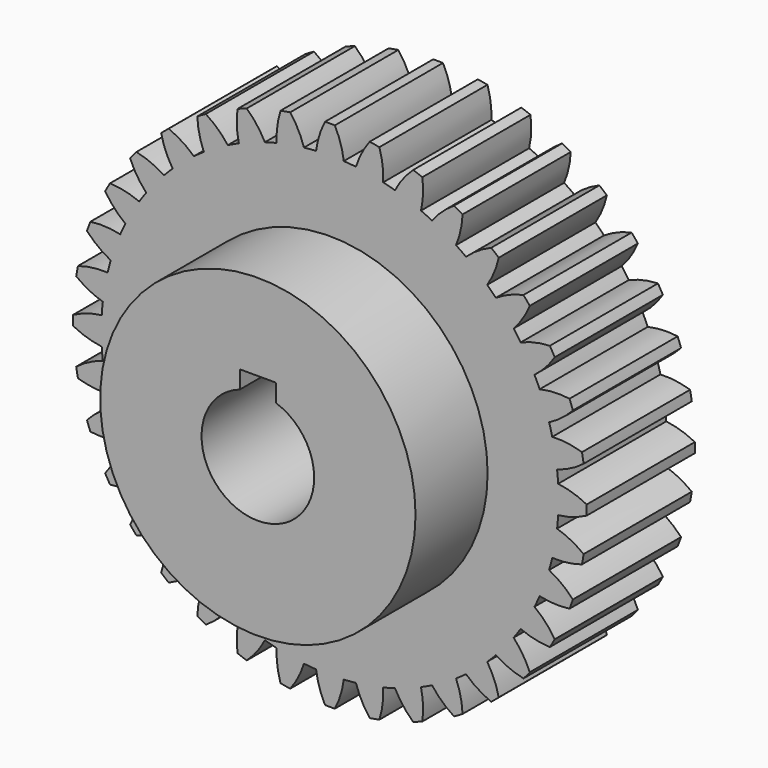
from build123d import *

# Parameters (mm, degrees)
F0_R     = 50.7435
F1_DEPTH = 30
F3_DEPTH = 30
F4_COUNT = 36
F5_R     = 35
F6_DEPTH = 20
F8_DEPTH = 50.001
F9_R     = 0.2


with BuildPart() as f1:
    # F0 (on Front) → F1 (new body)
    with BuildSketch(Plane.XZ):
        Circle(F0_R)
    extrude(amount=F1_DEPTH)

    # F2 (on Front) → F3 (join, through all)
    with BuildSketch(Plane.XZ):
        with BuildLine():
            ThreePointArc((-3.0719780243, 50.6504268814), (0, 50.7435), (3.0719780243, 50.6504268814))
            ThreePointArc((3.0719780243, 50.6504268814), (2.3675990404, 53.9099135714), (1.088572974, 56.9896043931))
            ThreePointArc((1.088572974, 56.9896043931), (0, 57), (-1.088572974, 56.9896043931))
            ThreePointArc((-1.088572974, 56.9896043931), (-2.3675990404, 53.9099135714), (-3.0719780243, 50.6504268814))
        make_face()
    extrude(amount=F3_DEPTH)

    # F4: F1 ×36 about axis
    f4_axis = Axis((0, 0, 0), (0, 1, 0))


with BuildPart() as f1_1:
    add(f1.part)
    for i in range(1, F4_COUNT):
        add(f1.part.rotate(f4_axis, i * 360 / F4_COUNT))

    # F5 (on face) → F6 (join)
    with BuildSketch(Plane.XZ.offset(30)):
        Circle(F5_R)
    extrude(amount=F6_DEPTH)

    # F7 (on Front) → F8 (cut, through all)
    with BuildSketch(Plane.XZ):
        with BuildLine():
            Line((4, 15.8), (-4, 15.8))
            Line((-4, 15.8), (-4, 11.8427192823))
            ThreePointArc((-4, 11.8427192823), (0, -12.5), (4, 11.8427192823))
            Line((4, 11.8427192823), (4, 15.8))
        make_face()
    extrude(amount=F8_DEPTH, mode=Mode.SUBTRACT)

    # F9
    f9_edges = [f1_1.edges().sort_by_distance(p)[0] for p in [
        (-4, -25, 15.8),
        (4, -25, 15.8),
    ]]
    fillet(f9_edges, radius=F9_R)


solid = f1_1.part
